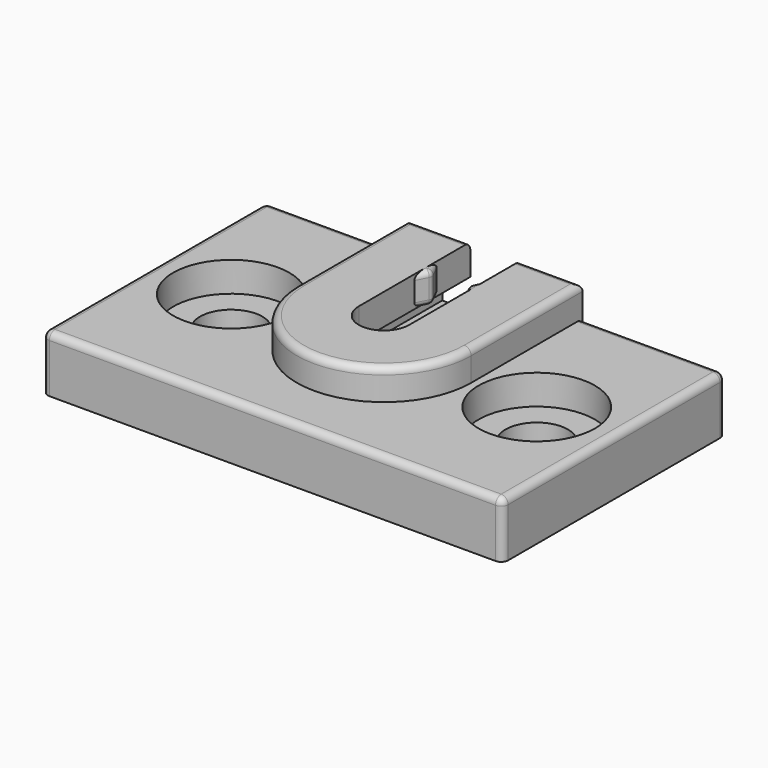
from build123d import *

# Parameters (mm, degrees)
F0_R     = 4.15
F1_DEPTH = 4
F0_R_2   = 2.225
F2_DEPTH = 1.87
F3_DEPTH = 6.2
F4_START = 4
F4_DEPTH = 2.2
F5_R     = 0.4
F6_R     = 0.5
F6_2_R   = 0.5


with BuildPart() as f1:
    # F0 (on Top) → F1 (new body)
    with BuildSketch(Plane.XY):
        with BuildLine():
            Line((-6.225, 9.95), (-16.425, 9.95))
            Line((-16.425, 9.95), (-16.425, -9.95))
            Line((-16.425, -9.95), (16.425, -9.95))
            Line((16.425, -9.95), (16.425, 9.95))
            Line((16.425, 9.95), (6.225, 9.95))
            Line((6.225, 9.95), (6.225, 0))
            ThreePointArc((6.225, 0), (0, -6.225), (-6.225, 0))
            Line((-6.225, 0), (-6.225, 9.95))
        make_face()
        with Locations((-10.905, 0)):
            Circle(F0_R, mode=Mode.SUBTRACT)
        with Locations((10.905, 0)):
            Circle(F0_R, mode=Mode.SUBTRACT)
    extrude(amount=F1_DEPTH)

    # F0 (on Top) → F2 (join)
    with BuildSketch(Plane.XY):
        with Locations((-10.905, 0)):
            Circle(F0_R)
        with Locations((-10.905, 0)):
            Circle(F0_R_2, mode=Mode.SUBTRACT)
        with Locations((10.905, 0)):
            Circle(F0_R)
        with Locations((10.905, 0)):
            Circle(F0_R_2, mode=Mode.SUBTRACT)
    extrude(amount=F2_DEPTH)

    # F6
    f6_edges = [f1.edges().sort_by_distance(p)[0] for p in [
        (0, -9.95, 4),
        (16.425, 0, 4),
        (-16.425, 0, 4),
        (-11.325, 9.95, 4),
        (11.325, 9.95, 4),
        (16.425, -9.95, 2),
        (-16.425, -9.95, 2),
        (16.425, 9.95, 2),
        (-16.425, 9.95, 2),
    ]]
    fillet(f6_edges, radius=F6_R)


with BuildPart() as f2:
    # F0 (on Top) → F2, piece 2 (new body)
    with BuildSketch(Plane.XY):
        with BuildLine():
            ThreePointArc((-1.8, 5.9590792074), (-2.8468319847, 5.5358985405), (-3.8, 4.9305805946))
            Line((-3.8, 4.9305805946), (-3.8, 0))
            ThreePointArc((-3.8, 0), (-3.2619012861, 1.949358869), (-1.8, 3.3466401061))
            Line((-1.8, 3.3466401061), (-1.8, 4.95))
            Line((-1.8, 4.95), (-1.8, 5.9590792074))
        make_face()
        with BuildLine():
            ThreePointArc((1.8, 3.3466401061), (0, 3.8), (-1.8, 3.3466401061))
            Line((-1.8, 3.3466401061), (-1.8, 0))
            ThreePointArc((-1.8, 0), (0, 1.8), (1.8, 0))
            Line((1.8, 0), (1.8, 3.3466401061))
        make_face()
        with BuildLine():
            ThreePointArc((-1.8, 3.3466401061), (-3.2619012861, 1.949358869), (-3.8, 0))
            ThreePointArc((-3.8, 0), (0, -3.8), (3.8, 0))
            ThreePointArc((3.8, 0), (3.2619012861, 1.949358869), (1.8, 3.3466401061))
            Line((1.8, 3.3466401061), (1.8, 0))
            ThreePointArc((1.8, 0), (0, -1.8), (-1.8, 0))
            Line((-1.8, 0), (-1.8, 3.3466401061))
        make_face()
        with BuildLine():
            ThreePointArc((1.8, 0), (0, 1.8), (-1.8, 0))
            ThreePointArc((-1.8, 0), (0, -1.8), (1.8, 0))
        make_face()
        with BuildLine():
            ThreePointArc((1.3620779041, 6.0741558083), (0, 6.225), (-1.3620779041, 6.0741558083))
            Line((-1.3620779041, 6.0741558083), (-1.3, 5.95))
            Line((-1.3, 5.95), (-1.8, 4.95))
            Line((-1.8, 4.95), (-1.8, 3.3466401061))
            ThreePointArc((-1.8, 3.3466401061), (0, 3.8), (1.8, 3.3466401061))
            Line((1.8, 3.3466401061), (1.8, 4.95))
            Line((1.8, 4.95), (1.3, 5.95))
            Line((1.3, 5.95), (1.3620779041, 6.0741558083))
        make_face()
        with BuildLine():
            Line((1.8, 9.95), (-1.8, 9.95))
            Line((-1.8, 9.95), (-1.8, 6.95))
            Line((-1.8, 6.95), (-1.3620779041, 6.0741558083))
            ThreePointArc((-1.3620779041, 6.0741558083), (0, 6.225), (1.3620779041, 6.0741558083))
            Line((1.3620779041, 6.0741558083), (1.8, 6.95))
            Line((1.8, 6.95), (1.8, 9.95))
        make_face()
        with BuildLine():
            Line((-1.8, 9.95), (-3.8, 9.95))
            Line((-3.8, 9.95), (-3.8, 4.9305805946))
            ThreePointArc((-3.8, 4.9305805946), (-2.8468319847, 5.5358985405), (-1.8, 5.9590792074))
            Line((-1.8, 5.9590792074), (-1.8, 6.95))
            Line((-1.8, 6.95), (-1.8, 9.95))
        make_face()
        with BuildLine():
            Line((3.8, 9.95), (1.8, 9.95))
            Line((1.8, 9.95), (1.8, 6.95))
            Line((1.8, 6.95), (1.8, 5.9590792074))
            ThreePointArc((1.8, 5.9590792074), (2.8468319847, 5.5358985405), (3.8, 4.9305805946))
            Line((3.8, 4.9305805946), (3.8, 9.95))
        make_face()
        with BuildLine():
            Line((3.8, 0), (3.8, 4.9305805946))
            ThreePointArc((3.8, 4.9305805946), (2.8468319847, 5.5358985405), (1.8, 5.9590792074))
            Line((1.8, 5.9590792074), (1.8, 4.95))
            Line((1.8, 4.95), (1.8, 3.3466401061))
            ThreePointArc((1.8, 3.3466401061), (3.2619012861, 1.949358869), (3.8, 0))
        make_face()
        with BuildLine():
            Line((1.8, 4.95), (1.8, 5.9590792074))
            ThreePointArc((1.8, 5.9590792074), (1.5820855931, 6.020600483), (1.3620779041, 6.0741558083))
            Line((1.3620779041, 6.0741558083), (1.3, 5.95))
            Line((1.3, 5.95), (1.8, 4.95))
        make_face()
        with BuildLine():
            Line((1.8, 5.9590792074), (1.8, 6.95))
            Line((1.8, 6.95), (1.3620779041, 6.0741558083))
            ThreePointArc((1.3620779041, 6.0741558083), (1.5820855931, 6.020600483), (1.8, 5.9590792074))
        make_face()
        with BuildLine():
            Line((-1.3620779041, 6.0741558083), (-1.8, 6.95))
            Line((-1.8, 6.95), (-1.8, 5.9590792074))
            ThreePointArc((-1.8, 5.9590792074), (-1.5820855931, 6.020600483), (-1.3620779041, 6.0741558083))
        make_face()
        with BuildLine():
            ThreePointArc((-1.3620779041, 6.0741558083), (-1.5820855931, 6.020600483), (-1.8, 5.9590792074))
            Line((-1.8, 5.9590792074), (-1.8, 4.95))
            Line((-1.8, 4.95), (-1.3, 5.95))
            Line((-1.3, 5.95), (-1.3620779041, 6.0741558083))
        make_face()
    extrude(amount=F2_DEPTH)


with BuildPart() as f3:
    # F0 (on Top) → F3 (new body)
    with BuildSketch(Plane.XY):
        with BuildLine():
            Line((-3.8, 9.95), (-6.225, 9.95))
            Line((-6.225, 9.95), (-6.225, 0))
            ThreePointArc((-6.225, 0), (-5.585947771, 2.7473282476), (-3.8, 4.9305805946))
            Line((-3.8, 4.9305805946), (-3.8, 9.95))
        make_face()
        with BuildLine():
            ThreePointArc((-3.8, 4.9305805946), (-5.585947771, 2.7473282476), (-6.225, 0))
            ThreePointArc((-6.225, 0), (0, -6.225), (6.225, 0))
            ThreePointArc((6.225, 0), (5.585947771, 2.7473282476), (3.8, 4.9305805946))
            Line((3.8, 4.9305805946), (3.8, 0))
            ThreePointArc((3.8, 0), (0, -3.8), (-3.8, 0))
            Line((-3.8, 0), (-3.8, 4.9305805946))
        make_face()
        with BuildLine():
            ThreePointArc((3.8, 4.9305805946), (5.585947771, 2.7473282476), (6.225, 0))
            Line((6.225, 0), (6.225, 9.95))
            Line((6.225, 9.95), (3.8, 9.95))
            Line((3.8, 9.95), (3.8, 4.9305805946))
        make_face()
    extrude(amount=F3_DEPTH)

    # F0 (on Top) → F4 (join)
    with BuildSketch(Plane.XY.offset(F4_START)):
        with BuildLine():
            Line((-1.8, 9.95), (-3.8, 9.95))
            Line((-3.8, 9.95), (-3.8, 4.9305805946))
            ThreePointArc((-3.8, 4.9305805946), (-2.8468319847, 5.5358985405), (-1.8, 5.9590792074))
            Line((-1.8, 5.9590792074), (-1.8, 6.95))
            Line((-1.8, 6.95), (-1.8, 9.95))
        make_face()
        with BuildLine():
            ThreePointArc((-1.8, 5.9590792074), (-2.8468319847, 5.5358985405), (-3.8, 4.9305805946))
            Line((-3.8, 4.9305805946), (-3.8, 0))
            ThreePointArc((-3.8, 0), (-3.2619012861, 1.949358869), (-1.8, 3.3466401061))
            Line((-1.8, 3.3466401061), (-1.8, 4.95))
            Line((-1.8, 4.95), (-1.8, 5.9590792074))
        make_face()
        with BuildLine():
            ThreePointArc((-1.8, 3.3466401061), (-3.2619012861, 1.949358869), (-3.8, 0))
            ThreePointArc((-3.8, 0), (0, -3.8), (3.8, 0))
            ThreePointArc((3.8, 0), (3.2619012861, 1.949358869), (1.8, 3.3466401061))
            Line((1.8, 3.3466401061), (1.8, 0))
            ThreePointArc((1.8, 0), (0, -1.8), (-1.8, 0))
            Line((-1.8, 0), (-1.8, 3.3466401061))
        make_face()
        with BuildLine():
            Line((3.8, 0), (3.8, 4.9305805946))
            ThreePointArc((3.8, 4.9305805946), (2.8468319847, 5.5358985405), (1.8, 5.9590792074))
            Line((1.8, 5.9590792074), (1.8, 4.95))
            Line((1.8, 4.95), (1.8, 3.3466401061))
            ThreePointArc((1.8, 3.3466401061), (3.2619012861, 1.949358869), (3.8, 0))
        make_face()
        with BuildLine():
            Line((3.8, 9.95), (1.8, 9.95))
            Line((1.8, 9.95), (1.8, 6.95))
            Line((1.8, 6.95), (1.8, 5.9590792074))
            ThreePointArc((1.8, 5.9590792074), (2.8468319847, 5.5358985405), (3.8, 4.9305805946))
            Line((3.8, 4.9305805946), (3.8, 9.95))
        make_face()
        with BuildLine():
            Line((-1.3620779041, 6.0741558083), (-1.8, 6.95))
            Line((-1.8, 6.95), (-1.8, 5.9590792074))
            ThreePointArc((-1.8, 5.9590792074), (-1.5820855931, 6.020600483), (-1.3620779041, 6.0741558083))
        make_face()
        with BuildLine():
            ThreePointArc((-1.3620779041, 6.0741558083), (-1.5820855931, 6.020600483), (-1.8, 5.9590792074))
            Line((-1.8, 5.9590792074), (-1.8, 4.95))
            Line((-1.8, 4.95), (-1.3, 5.95))
            Line((-1.3, 5.95), (-1.3620779041, 6.0741558083))
        make_face()
        with BuildLine():
            Line((1.8, 4.95), (1.8, 5.9590792074))
            ThreePointArc((1.8, 5.9590792074), (1.5820855931, 6.020600483), (1.3620779041, 6.0741558083))
            Line((1.3620779041, 6.0741558083), (1.3, 5.95))
            Line((1.3, 5.95), (1.8, 4.95))
        make_face()
        with BuildLine():
            Line((1.8, 5.9590792074), (1.8, 6.95))
            Line((1.8, 6.95), (1.3620779041, 6.0741558083))
            ThreePointArc((1.3620779041, 6.0741558083), (1.5820855931, 6.020600483), (1.8, 5.9590792074))
        make_face()
    extrude(amount=F4_DEPTH)

    # F5
    f5_edges = [f3.edges().sort_by_distance(p)[0] for p in [
        (1.55, 6.45, 6.2),
        (1.55, 5.45, 6.2),
        (-1.55, 5.45, 6.2),
        (-1.55, 6.45, 6.2),
        (-1.55, 6.45, 4),
        (1.55, 6.45, 4),
        (-1.55, 5.45, 4),
        (1.55, 5.45, 4),
        (-1.3, 5.95, 5.1),
        (1.3, 5.95, 5.1),
    ]]
    fillet(f5_edges, radius=F5_R)

    # F6#2
    f6_2_edges = [f3.edges().sort_by_distance(p)[0] for p in [
        (-4.0125, 9.95, 6.2),
        (4.0125, 9.95, 6.2),
        (6.225, 4.975, 6.2),
    ]]
    fillet(f6_2_edges, radius=F6_2_R)


solid = Compound([f1.part, f2.part, f3.part])
